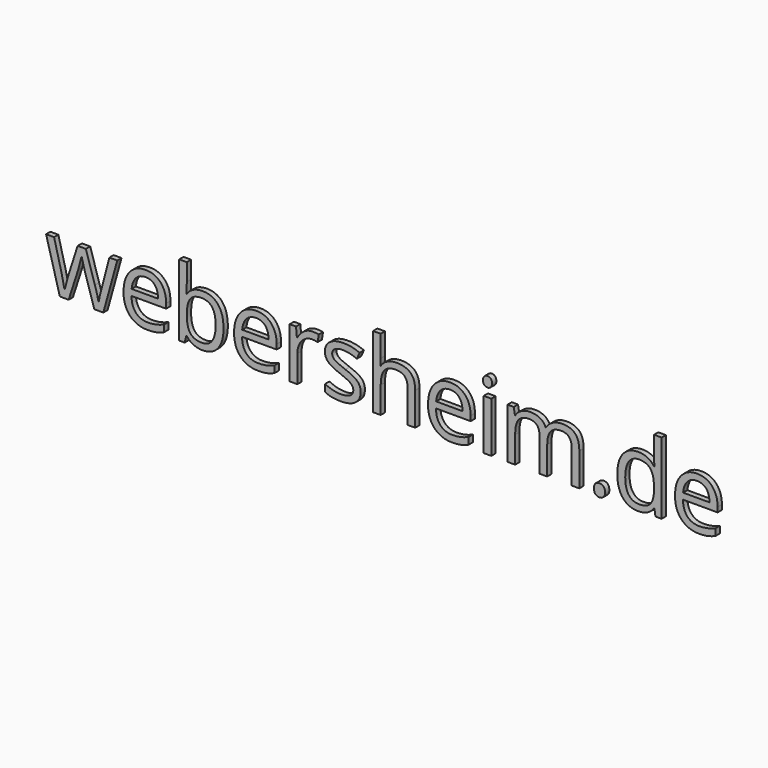
from build123d import *

# Parameters (mm, degrees)
F0_TEXT_SIZE = 35.0921026741
F1_DEPTH     = 2


# Not quite as in the source:
# - Text() gives the source's letters only with a copy of the font that has no kerning and outlines rounded to 1/6400 em; it was checked with that copy


with BuildPart() as f1:
    # F0 (on Front) → F1 (new body)
    with BuildSketch(Plane.XZ):
        with Locations((-60.5689734221, 10.7381846756)):
            Text('webersheim.de', F0_TEXT_SIZE, font='Open Sans', text_align=(TextAlign.LEFT, TextAlign.BOTTOM))
    extrude(amount=F1_DEPTH)


solid = f1.part
